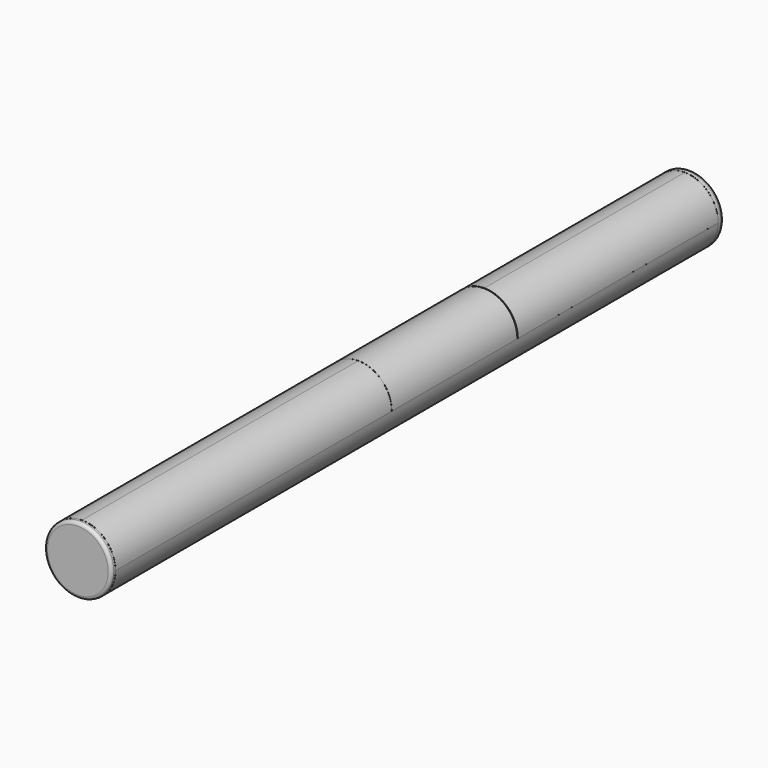
from build123d import *

# Parameters (mm, degrees)
F1_DEPTH  = 180
F3_DEPTH  = 120
F4_R      = 16
F5_DEPTH  = 3.5
F8_R      = 2
F10_R     = 16
F11_DEPTH = 2.5
F15_R     = 1.5
F19_DEPTH = 82.5
F26_DEPTH = 10
F30_DEPTH = 75
F36_W     = 21
F36_H     = 2
F37_DEPTH = 2


with BuildPart() as f1:
    # F0 (on Front) → F1 (new body, symmetric)
    with BuildSketch(Plane.XZ):
        with BuildLine():
            Line((0, -8.884137), (0, -16))
            ThreePointArc((0, -16), (11.313708, -11.313708), (16, 0))
            Line((16, 0), (12.75, 0))
            Line((12.75, 0), (12.75, 2.1))
            Line((12.75, 2.1), (14.25, 2.1))
            Line((14.25, 2.1), (14.25, 4.1))
            Line((14.25, 4.1), (10.5, 4.1))
            Line((10.5, 4.1), (10.5, -1.9))
            Line((10.5, -1.9), (6.5, -1.9))
            Line((6.5, -1.9), (6.5, -4.9))
            Line((6.5, -4.9), (0, -8.884137))
        make_face()
        with BuildLine():
            ThreePointArc((-16, 0), (-11.313708, -11.313708), (0, -16))
            Line((0, -16), (0, -8.884137))
            Line((0, -8.884137), (-6.5, -4.9))
            Line((-6.5, -4.9), (-6.5, -1.9))
            Line((-6.5, -1.9), (-10.5, -1.9))
            Line((-10.5, -1.9), (-10.5, 4.1))
            Line((-10.5, 4.1), (-14.25, 4.1))
            Line((-14.25, 4.1), (-14.25, 2.1))
            Line((-14.25, 2.1), (-12.75, 2.1))
            Line((-12.75, 2.1), (-12.75, 0))
            Line((-12.75, 0), (-16, 0))
        make_face()
    extrude(amount=F1_DEPTH, both=True)


with BuildPart() as f3:
    # F2 (on Front) → F3 (new body)
    with BuildSketch(Plane.XZ):
        with BuildLine():
            Line((12.933292, 6.649997), (15.999999, 6.649997))
            ThreePointArc((15.999999, 6.649997), (11.313708, 17.963706), (-1e-06, 22.649997))
            Line((-1e-06, 22.649997), (-1e-06, 21.149997))
            ThreePointArc((-1e-06, 21.149997), (8.620469, 18.309221), (13.86317, 10.899997))
            Line((13.86317, 10.899997), (14.46317, 10.899997))
            Line((14.46317, 10.899997), (14.46317, 8.649997))
            Line((14.46317, 8.649997), (12.933292, 8.649997))
            Line((12.933292, 8.649997), (12.933292, 6.649997))
        make_face()
        with BuildLine():
            Line((-1e-06, 21.149997), (-1e-06, 22.649997))
            ThreePointArc((-1e-06, 22.649997), (-11.313709, 17.963706), (-16.000001, 6.649997))
            Line((-16.000001, 6.649997), (-12.933294, 6.649997))
            Line((-12.933294, 6.649997), (-12.933294, 8.649997))
            Line((-12.933294, 8.649997), (-14.463171, 8.649997))
            Line((-14.463171, 8.649997), (-14.463171, 10.899997))
            Line((-14.463171, 10.899997), (-13.863171, 10.899997))
            ThreePointArc((-13.863171, 10.899997), (-8.620471, 18.309221), (-1e-06, 21.149997))
        make_face()
    extrude(amount=F3_DEPTH)


with BuildPart() as f5:
    # F4 (on Front) → F5 (new body)
    with BuildSketch(Plane.XZ):
        with Locations((33.5, 0)):
            Circle(F4_R)
    extrude(amount=F5_DEPTH)


with BuildPart() as f6_1:
    # F6: copy of F3
    add(f3.part.moved(Location((0, 155, 0))))


with BuildPart() as f5_1:
    # F7: moved
    add(f5.part.moved(Location((-33.5, 184.33, 0))))

    # F8
    f8_edges = [f5_1.edges().sort_by_distance(p)[0] for p in [
        (-16, 184.33, 0),
    ]]
    fillet(f8_edges, radius=F8_R)


with BuildPart() as f5_2:
    # F9: moved
    add(f5_1.part.moved(Location((0, -0.8, 0))))


with BuildPart() as f11:
    # F10 (on Front) → F11 (new body)
    with BuildSketch(Plane.XZ):
        with Locations((33.5, 0)):
            Circle(F10_R)
    extrude(amount=F11_DEPTH)


with BuildPart() as f11_1:
    # F12: moved
    add(f11.part.moved(Location((0, -180, 0))))


with BuildPart() as f3_1:
    # F13: moved
    add(f3.part.moved(Location((0, -30, -6.7))))


with BuildPart() as f11_2:
    # F14: moved
    add(f11_1.part.moved(Location((-33.5, 0, 0))))

    # F15
    f15_edges = [f11_2.edges().sort_by_distance(p)[0] for p in [
        (-16, -182.5, 0),
    ]]
    fillet(f15_edges, radius=F15_R)


with BuildPart() as f16_1:
    # F16: copy of F3
    add(f3_1.part.moved(Location((0, 210.3, 0))))


with BuildPart() as f19:
    # F18 (on Front) → F19 (new body, symmetric)
    with BuildSketch(Plane.XZ):
        with BuildLine():
            ThreePointArc((15.999999, 28.000001), (11.313708, 39.313709), (-1e-06, 44.000001))
            Line((-1e-06, 44.000001), (-1e-06, 42.500001))
            ThreePointArc((-1e-06, 42.500001), (8.63985, 39.64487), (13.877231, 32.203859))
            Line((13.877231, 32.203859), (14.477231, 32.203859))
            Line((14.477231, 32.203859), (14.489533, 29.953893))
            Line((14.489533, 29.953893), (12.989556, 29.945692))
            Line((12.989556, 29.945692), (13.00049, 27.945722))
            Line((13.00049, 27.945722), (15.999999, 28.000001))
        make_face()
        with BuildLine():
            Line((-1e-06, 42.500001), (-1e-06, 44.000001))
            ThreePointArc((-1e-06, 44.000001), (-11.313709, 39.313709), (-16.000001, 28.000001))
            Line((-16.000001, 28.000001), (-13.000492, 27.945722))
            Line((-13.000492, 27.945722), (-12.989557, 29.945692))
            Line((-12.989557, 29.945692), (-14.489535, 29.953893))
            Line((-14.489535, 29.953893), (-14.477233, 32.203859))
            Line((-14.477233, 32.203859), (-13.877233, 32.203859))
            ThreePointArc((-13.877233, 32.203859), (-8.639852, 39.64487), (-1e-06, 42.500001))
        make_face()
    extrude(amount=F19_DEPTH, both=True)


with BuildPart() as f19_1:
    # F20: moved
    add(f19.part.moved(Location((0, 90, -28))))


with BuildPart() as f19_2:
    # F22: moved
    add(f19_1.part.moved(Location((0, -149.5, 0))))


with BuildPart() as f11_3:
    # F23: moved
    add(f11_2.part.moved(Location((0, -45.1, 0))))


with BuildPart() as f19_3:
    # F24: moved
    add(f19_2.part.moved(Location((0, -45.55, 0))))


with BuildPart() as f26:
    # F25 (on Front) → F26 (new body)
    with BuildSketch(Plane.XZ):
        Polygon((-6.397317, -3.548501), (-6.402676, -4.798489), (0, -8.704349), (6.402683, -4.798501), (6.402683, -3.548501), align=None)
    extrude(amount=F26_DEPTH)


with BuildPart() as f26_1:
    # F27: moved
    add(f26.part.moved(Location((0, -172, 0))))


with BuildPart() as f28_1:
    # F28: copy of F26
    add(f26_1.part.moved(Location((0, 354, 0))))


with BuildPart() as f30:
    # F29 (on Front) → F30 (new body)
    with BuildSketch(Plane.XZ):
        with BuildLine():
            Line((12.5, 12), (16, 12))
            ThreePointArc((16, 12), (0, 28), (-16, 12))
            Line((-16, 12), (-12.5, 12))
            ThreePointArc((-12.5, 12), (0, 24.5), (12.5, 12))
        make_face()
    extrude(amount=F30_DEPTH)


with BuildPart() as f30_1:
    # F31: moved
    add(f30.part.moved(Location((0, 15, -12))))


with BuildPart() as f19_4:
    # F32: moved
    add(f19_3.part.moved(Location((0, -15, 0))))


with BuildPart() as f30_2:
    # F33: moved
    add(f30_1.part.moved(Location((0, 45, 0))))


with BuildPart() as f19_5:
    # F34: moved
    add(f19_4.part.moved(Location((0, 45, 0))))


with BuildPart() as f19_6:
    # F35: moved
    add(f19_5.part.moved(Location((0, -22.5, 0))))


with BuildPart() as f37:
    # F36 (on Front) → F37 (new body)
    with BuildSketch(Plane.XZ):
        with Locations((-0.053476, 8.999999)):
            Rectangle(F36_W, F36_H)
    extrude(amount=F37_DEPTH)


with BuildPart() as f37_1:
    # F38: moved
    add(f37.part.moved(Location((0, -178, -9.9))))


with BuildPart() as f39_1:
    # F39: copy of F37
    add(f37_1.part.moved(Location((0, 358, 0))))


with BuildPart() as f11_4:
    # F40: moved
    add(f11_3.part.moved(Location((0, 45, 0))))


solid = Compound([f1.part, f5_2.part, f16_1.part, f26_1.part, f28_1.part, f30_2.part, f19_6.part, f37_1.part, f39_1.part, f11_4.part])
